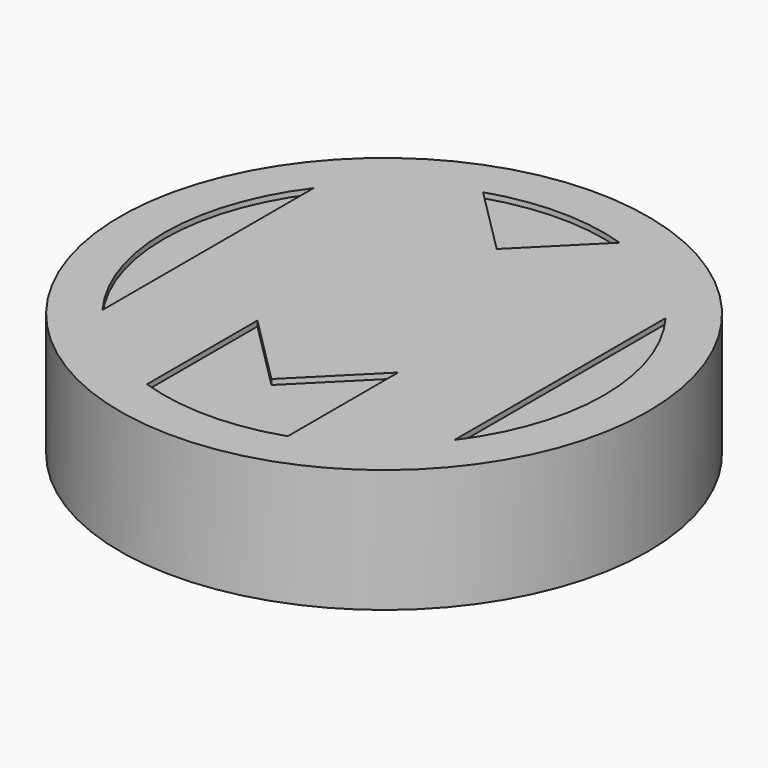
from build123d import *

# Parameters (mm, degrees)
F0_R            = 38.1
F0_R_2          = 34.29
F1_DEPTH        = 7.62
F2_DEPTH        = 17.78
F4_DEPTH        = 10.16
F5_DEPTH        = 10.16
F5_COPIES_COUNT = 4
F6_DEPTH        = 10.16
F6_COPIES_COUNT = 8
F8_DEPTH        = 0.762


# Not quite as in the source:
# - a pattern or mirror of a feature is missing from the dataset's text; its kind, count and spacing are read off the source's solid


with BuildPart() as f1:
    # F0 (on Top) → F1 (new body)
    with BuildSketch(Plane.XY):
        Circle(F0_R)
        Circle(F0_R_2, mode=Mode.SUBTRACT)
        Circle(F0_R_2)
    extrude(amount=-F1_DEPTH)

    # F0 (on Top) → F2 (join)
    with BuildSketch(Plane.XY):
        Circle(F0_R)
        Circle(F0_R_2, mode=Mode.SUBTRACT)
    extrude(amount=-F2_DEPTH)

    # F3 (on face) → F4 (join)
    with BuildSketch(Plane(origin=(0, 0, -7.62), x_dir=(1, 0, 0), z_dir=(0, 0, -1))):
        with BuildLine():
            Line((-4.7088706862, -3.0087008594), (-0.9977636205, -2.3358227154))
            ThreePointArc((-0.9977636205, -2.3358227154), (0, -2.54), (0.9977636205, -2.3358227154))
            Line((0.9977636205, -2.3358227154), (4.7088706862, -3.0087008594))
            Line((4.7088706862, -3.0087008594), (2.5217636205, 0.3038227154))
            ThreePointArc((2.5217636205, 0.3038227154), (2.1997045256, 1.27), (1.524, 2.032))
            Line((1.524, 2.032), (0, 5.588))
            Line((0, 5.588), (-1.524, 2.032))
            ThreePointArc((-1.524, 2.032), (-2.1997045256, 1.27), (-2.5217636205, 0.3038227154))
            Line((-2.5217636205, 0.3038227154), (-4.7088706862, -3.0087008594))
        make_face()
    extrude(amount=F4_DEPTH)

    # F3 (on face) → F5 (join)
    with BuildSketch(Plane(origin=(0, 0, -7.62), x_dir=(1, 0, 0), z_dir=(0, 0, -1))):
        Polygon((3.81, 14.9225), (0, 17.7165), (-3.81, 14.9225), (0, 12.1285), align=None)
    f5 = extrude(amount=F5_DEPTH)

    # F5_copies: F5 ×4 about axis
    f5_copies_axis = Axis((0, 0, 0), (0, 0, 1))
    for i in range(1, F5_COPIES_COUNT):
        add(f5.rotate(f5_copies_axis, i * 360 / F5_COPIES_COUNT))

    # F3 (on face) → F6 (join)
    with BuildSketch(Plane(origin=(0, 0, -7.62), x_dir=(1, 0, 0), z_dir=(0, 0, -1))):
        Polygon((3.81, 26.7335), (0, 29.5275), (-3.81, 26.7335), (0, 23.9395), align=None)
    f6 = extrude(amount=F6_DEPTH)

    # F6_copies: F6 ×8 about axis
    f6_copies_axis = Axis((0, 0, 0), (0, 0, 1))
    for i in range(1, F6_COPIES_COUNT):
        add(f6.rotate(f6_copies_axis, i * 360 / F6_COPIES_COUNT))

    # F7 (on face) → F8 (cut)
    with BuildSketch(Plane.XY):
        with BuildLine():
            Line((-10.16, -10.16), (-10.16, -30.0805069771))
            ThreePointArc((-10.16, -30.0805069771), (0, -31.75), (10.16, -30.0805069771))
            Line((10.16, -30.0805069771), (10.16, -10.16))
            Line((10.16, -10.16), (0, -20.32))
            Line((0, -20.32), (-10.16, -10.16))
        make_face()
        with BuildLine():
            ThreePointArc((-25.4, 19.05), (-31.75, 0), (-25.4, -19.05))
            Line((-25.4, -19.05), (-25.4, 19.05))
        make_face()
        with BuildLine():
            ThreePointArc((25.4, -19.05), (31.75, 0), (25.4, 19.05))
            Line((25.4, 19.05), (25.4, -19.05))
        make_face()
        with BuildLine():
            ThreePointArc((9.8601311185, 30.1801311185), (0, 31.75), (-9.8601311185, 30.1801311185))
            Line((-9.8601311185, 30.1801311185), (0, 20.32))
            Line((0, 20.32), (9.8601311185, 30.1801311185))
        make_face()
    extrude(amount=-F8_DEPTH, mode=Mode.SUBTRACT)


solid = f1.part
